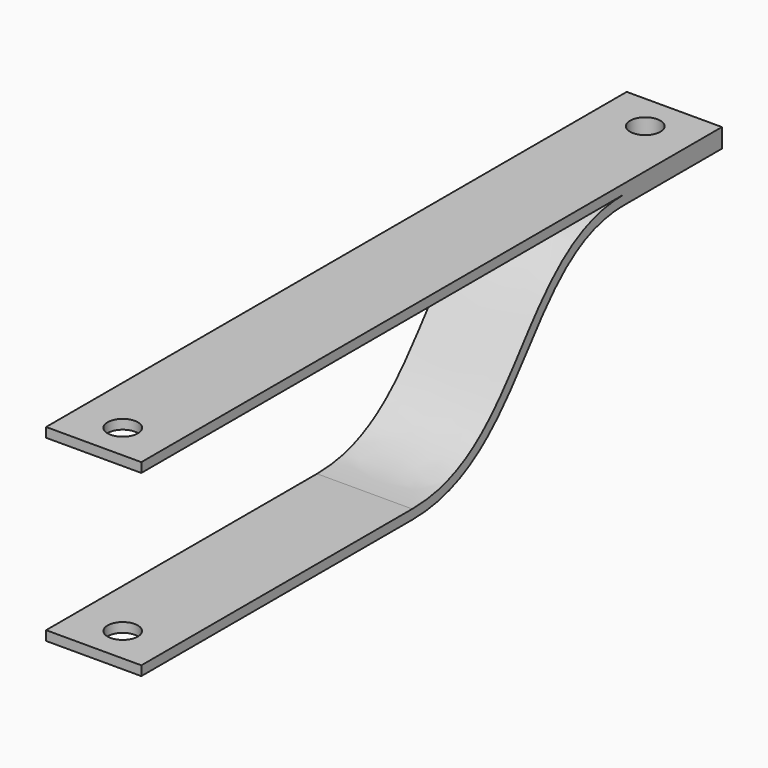
from build123d import *

# Parameters (mm, degrees)
F1_DEPTH = 50
F2_R     = 7.9375
F3_DEPTH = 98.9010001


# Not quite as in the source:
# - the dataset's text gives a spline's control points without its knots; the knots are read off the source's solid


with BuildPart() as f1:
    # F0 (on Right) → F1 (new body)
    with BuildSketch(Plane.YZ):
        Polygon((0, 5), (0, 0), (317.0611265182, 0), (381, 0), (381, 5), align=None)
        with BuildLine():
            Line((381, 0), (317.0611265182, 0))
            add(Edge.make_bspline(
                [(177.8, -88.9), (248.9784660816, -88.9), (248.9784660816, 0), (317.0611265182, 0)],
                knots=[0, 0, 0, 0, 165.2176484493, 165.2176484493, 165.2176484493, 165.2176484493], degree=3))
            Line((177.8, -88.9), (0, -88.9))
            Line((0, -88.9), (0, -93.9))
            Line((0, -93.9), (177.8, -93.9))
            add(Edge.make_bspline(
                [(177.8, -93.9), (182.5088568902, -93.9), (191.4045001846, -93.163983571), (203.303724493, -90.0815735434), (213.8561143205, -85.3057917839), (223.1918502865, -79.1733759879), (231.500279729, -72.0263439941), (241.5096982859, -61.5630106154), (252.6106670588, -47.4521159829), (263.297288811, -33.7461247303), (272.3524018342, -24.0513036385), (279.564351284, -17.6529202199), (287.3719173686, -12.3368323414), (295.9847641829, -8.2781357767), (305.6793231482, -5.6490337962), (313.0779947533, -5), (317.0611265182, -5)],
                knots=[0, 0, 0, 0, 0.0625, 0.125, 0.1875, 0.25, 0.3125, 0.375, 0.5, 0.625, 0.6875, 0.75, 0.8125, 0.875, 0.9375, 1, 1, 1, 1], degree=3))
            Line((317.0611265182, -5), (381, -5))
            Line((381, -5), (381, 0))
        make_face()
    extrude(amount=-F1_DEPTH)

    # F2 (on face) → F3 (cut, through all)
    with BuildSketch(Plane.XY.offset(5)):
        with Locations((-25, 361.95)):
            Circle(F2_R)
        with Locations((-25, 19.05)):
            Circle(F2_R)
    extrude(amount=-F3_DEPTH, mode=Mode.SUBTRACT)


solid = f1.part
